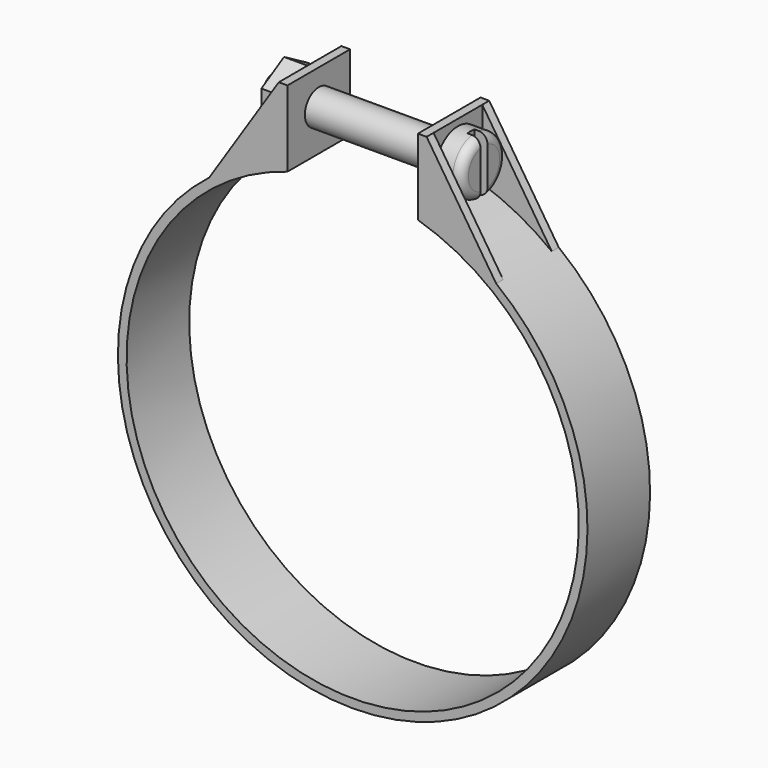
from build123d import *

# Parameters (mm, degrees)
F1_DEPTH         = 4.5
F3_DEPTH         = 1
F3_COPIES2_COUNT = 2
F5_DEPTH         = 3
F6_R             = 3.25
F7_DEPTH         = 3
F8_R             = 2
F9_DEPTH         = 20
F10_W            = 1
F10_H            = 6.5
F11_DEPTH        = 1.5
F12_R            = 1


# Not quite as in the source:
# - a pattern or mirror of a feature is missing from the dataset's text; its kind, count and spacing are read off the source's solid


with BuildPart() as f1:
    # F0 (on Front) → F1 (new body, symmetric)
    with BuildSketch(Plane.XZ):
        with BuildLine():
            Line((-8.5, 33.6271340575), (-8.5, 25.6271340575))
            ThreePointArc((-8.5, 25.6271340575), (0, -27), (8.5, 25.6271340575))
            Line((8.5, 25.6271340575), (8.5, 33.6271340575))
            Line((8.5, 33.6271340575), (7.5, 33.6271340575))
            Line((7.5, 33.6271340575), (7.5, 24.894778569))
            ThreePointArc((7.5, 24.894778569), (0, -26), (-7.5, 24.894778569))
            Line((-7.5, 24.894778569), (-7.5, 33.6271340575))
            Line((-7.5, 33.6271340575), (-8.5, 33.6271340575))
        make_face()
    extrude(amount=F1_DEPTH, both=True)

    # F2 (on face) → F3 (join)
    with BuildSketch(Plane.XZ.offset(4.5)):
        with BuildLine():
            Line((-8.5, 25.6271340575), (-8.5, 33.6271340575))
            Line((-8.5, 33.6271340575), (-16.5, 21.3717102732))
            ThreePointArc((-16.5, 21.3717102732), (-12.6797932907, 23.8374252407), (-8.5, 25.6271340575))
        make_face()
    f3 = extrude(amount=-F3_DEPTH)

    # F3_copies: F3 across plane
    add(f3.mirror(Plane.ZX))

    # F3_copies1: F3 across plane
    add(f3.mirror(Plane(origin=(0, 0, 0), x_dir=(0, 0, 1), z_dir=(1, 0, 0))))

    # F3_copies2: F3 ×2 about axis
    f3_copies2_axis = Axis((0, 0, 0), (0, 0, 1))
    for i in range(1, F3_COPIES2_COUNT):
        add(f3.rotate(f3_copies2_axis, i * 360 / F3_COPIES2_COUNT))

    # F4 (on face) → F5 (join)
    with BuildSketch(Plane(origin=(-8.5, 0, 0), x_dir=(0, -1, 0), z_dir=(-1, 0, 0))):
        Polygon((-3.25, 31.5035224323), (-3.25, 27.7507456826), (0, 25.8743573077), (3.25, 27.7507456826), (3.25, 31.5035224323), (0, 33.3799108072), align=None)
    extrude(amount=F5_DEPTH)

    # F6 (on face) → F7 (join)
    with BuildSketch(Plane.YZ.offset(8.5)):
        with Locations((0, 29.6271340575)):
            Circle(F6_R)
    extrude(amount=F7_DEPTH)

    # F8 (on face) → F9 (join)
    with BuildSketch(Plane(origin=(7.5, 0, 0), x_dir=(0, -1, 0), z_dir=(-1, 0, 0))):
        with Locations((0, 29.6271340575)):
            Circle(F8_R)
    extrude(amount=F9_DEPTH)

    # F10 (on face) → F11 (cut)
    with BuildSketch(Plane.YZ.offset(11.5)):
        with Locations((0, 29.6271340575)):
            Rectangle(F10_W, F10_H)
    extrude(amount=-F11_DEPTH, mode=Mode.SUBTRACT)

    # F12
    f12_edges = [f1.edges().sort_by_distance(p)[0] for p in [
        (11.5, -3.25, 29.627134),
        (11.5, 2.468552, 31.741076),
        (11.5, 2.468552, 27.513192),
    ]]
    fillet(f12_edges, radius=F12_R)


solid = f1.part
